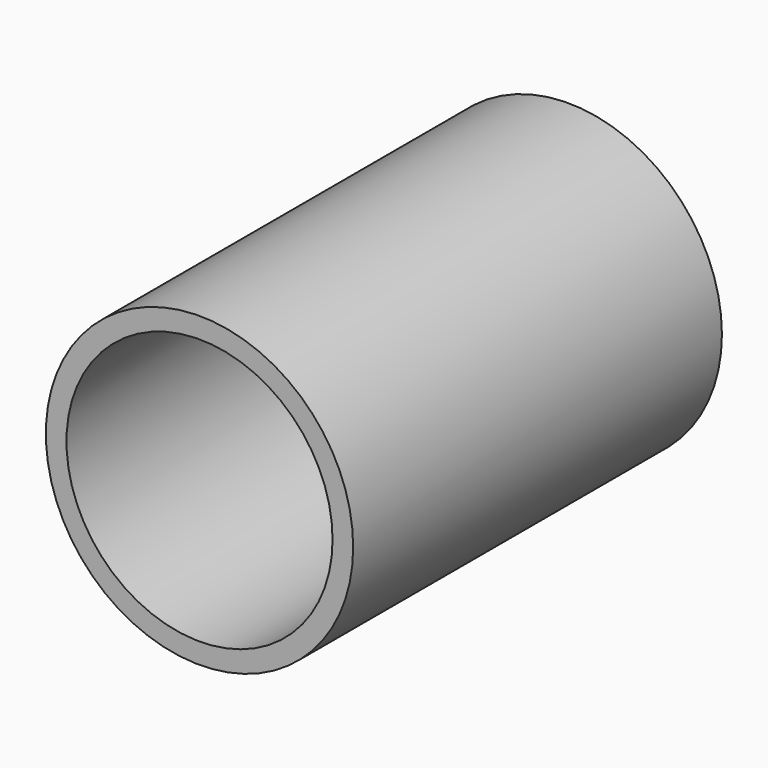
from build123d import *

# Parameters (mm, degrees)
F0_R     = 50.8
F1_DEPTH = 152.4
F2_R     = 43.9882205893
F3_DEPTH = 127


# Not quite as in the source:
# - a feature names something its author has since deleted; it is built from what else it names


with BuildPart() as f1:
    # F0 (on Front) → F1 (new body)
    with BuildSketch(Plane.XZ):
        Circle(F0_R)
    extrude(amount=F1_DEPTH)

    # F2 (on face) → F3 (cut)
    with BuildSketch(Plane.XZ.offset(152.4)):
        Circle(F2_R)
    extrude(amount=-F3_DEPTH, mode=Mode.SUBTRACT)


solid = f1.part
